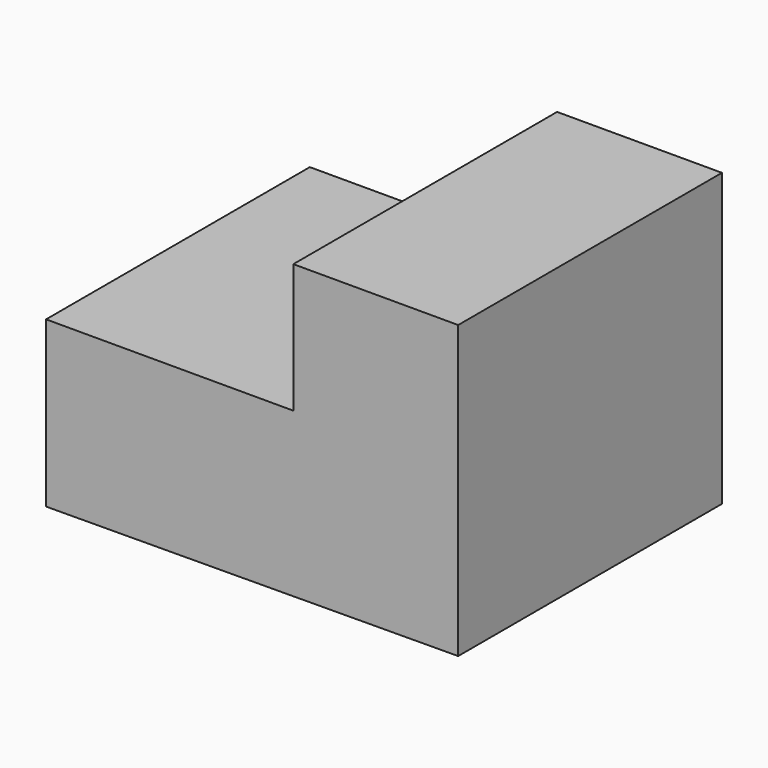
from build123d import *

# Parameters (mm, degrees)
F1_DEPTH = 25.4


# Not quite as in the source:
# - a feature names something its author has since deleted; it is built from what else it names


with BuildPart() as f1:
    # F0 (on Front) → F1 (new body)
    with BuildSketch(Plane.XZ):
        Polygon((-48.536748241, -30.1682058325), (-48.536748241, -42.8682058325), (-16.786748241, -42.6841488952), (-16.786748241, -20.229075549), (-29.486748241, -20.229075549), (-29.486748241, -30.1682058325), align=None)
    extrude(amount=F1_DEPTH)


solid = f1.part
